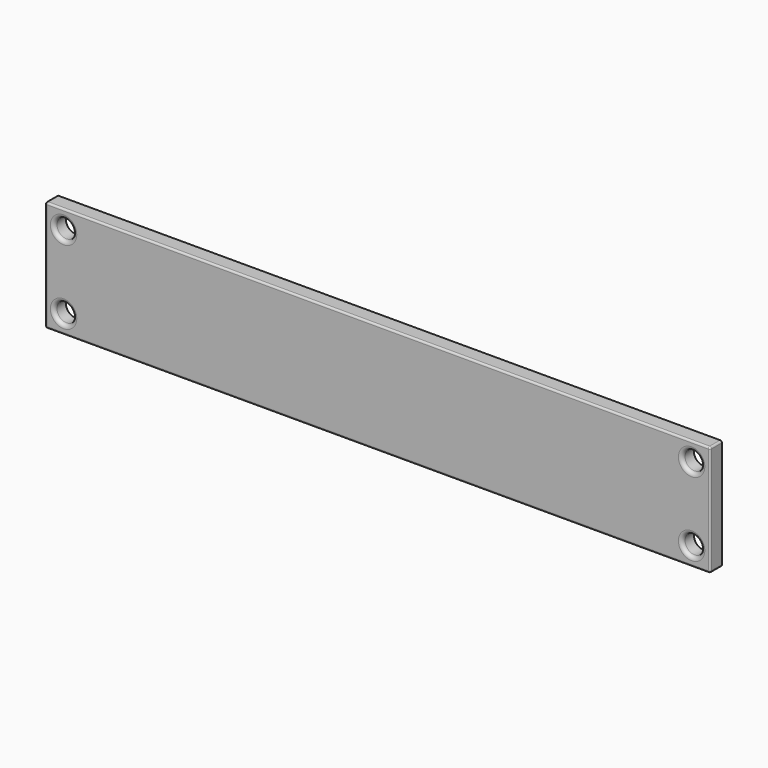
from build123d import *

# Parameters (mm, degrees)
F0_W         = 180
F0_H         = 30
F0_R         = 2.5751263091
F1_DEPTH     = 4
F2_R         = 1
F3_R         = 0.5
F4_TEXT_SIZE = 10.7463689027
F5_DEPTH     = 1


# Not quite as in the source:
# - a feature names something its author has since deleted; it is built from what else it names
# - Text() gives the source's letters only with a copy of the font that has no kerning and outlines rounded to 1/6400 em; it was checked with that copy


with BuildPart() as f1:
    # F0 (on Front) → F1 (new body)
    with BuildSketch(Plane.XZ):
        Rectangle(F0_W, F0_H)
        with Locations((-85, -10)):
            Circle(F0_R, mode=Mode.SUBTRACT)
        with Locations((85, -10)):
            Circle(F0_R, mode=Mode.SUBTRACT)
        with Locations((-85, 10)):
            Circle(F0_R, mode=Mode.SUBTRACT)
        with Locations((85, 10)):
            Circle(F0_R, mode=Mode.SUBTRACT)
    extrude(amount=F1_DEPTH)

    # F2
    f2_edges = [f1.edges().sort_by_distance(p)[0] for p in [
        (-87.575126, -4, 10),
        (-87.575126, -4, -10),
        (82.424874, -4, 10),
        (82.424874, -4, -10),
    ]]
    fillet(f2_edges, radius=F2_R)

    # F3
    f3_edges = [f1.edges().sort_by_distance(p)[0] for p in [
        (0, -4, 15),
        (-90, -4, 0),
        (0, -4, -15),
        (90, -4, 0),
        (-90, -2, 15),
        (-90, -2, -15),
        (90, -2, 15),
        (90, -2, -15),
    ]]
    fillet(f3_edges, radius=F3_R)

    # F4 (on face) → F5 (join)
    with BuildSketch(Plane(origin=(0, 0, 0), x_dir=(-1, 0, 0), z_dir=(0, 1, 0))):
        with Locations((-69.5098517463, -4.47527963)):
            Text('Berea FP RB', F4_TEXT_SIZE, font='Open Sans', text_align=(TextAlign.LEFT, TextAlign.BOTTOM))
    extrude(amount=F5_DEPTH)

    # F6: F1 across plane


with BuildPart() as f1_1:
    add(f1.part)
    add(f1.part.mirror(Plane.YZ))


solid = f1_1.part
